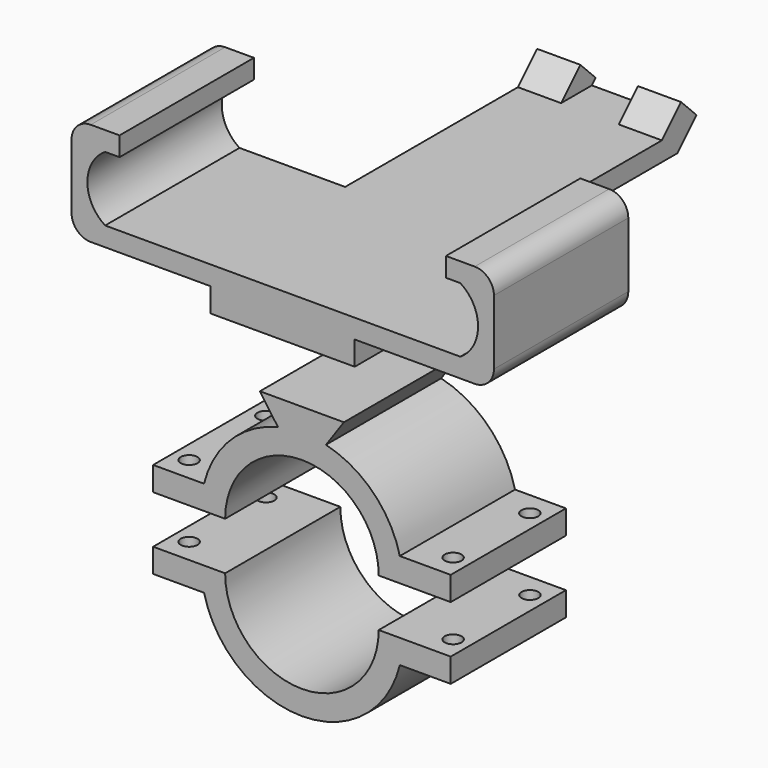
from build123d import *

# Parameters (mm, degrees)
F3_DEPTH      = 30
F4_DEPTH      = 5
F6_DEPTH      = 15
F6_DEPTH_BACK = 15
F7_DEPTH      = 6
F8_DEPTH      = 30
F9_DEPTH      = 30
F10_R         = 1.75
F11_DEPTH     = 50


# Not quite as in the source:
# - a feature names something its author has since deleted; it is built from what else it names


with BuildPart() as f3:
    # F2 (on offset) → F3 (new body)
    with BuildSketch(Plane.XZ.offset(30)):
        with BuildLine():
            Line((37, 49), (-37, 49))
            ThreePointArc((-37, 49), (-40.7061089907, 55.75), (-37, 62.5))
            Line((-37, 62.5), (-34, 62.5))
            Line((-34, 62.5), (-34, 66.5))
            Line((-34, 66.5), (-40, 66.5))
            ThreePointArc((-40, 66.5), (-42.8284271247, 65.3284271247), (-44, 62.5))
            Line((-44, 62.5), (-44, 49))
            ThreePointArc((-44, 49), (-42.8284271247, 46.1715728753), (-40, 45))
            Line((-40, 45), (-15, 45))
            Line((-15, 45), (-15, 40))
            Line((-15, 40), (-5.798962309, 40))
            Line((-5.798962309, 40), (-9.3, 45))
            Line((-9.3, 45), (9.3, 45))
            Line((9.3, 45), (5.798962309, 40))
            Line((5.798962309, 40), (15, 40))
            Line((15, 40), (15, 45))
            Line((15, 45), (40, 45))
            ThreePointArc((40, 45), (42.8284271247, 46.1715728753), (44, 49))
            Line((44, 49), (44, 62.5))
            ThreePointArc((44, 62.5), (42.8284271247, 65.3284271247), (40, 66.5))
            Line((40, 66.5), (34, 66.5))
            Line((34, 66.5), (34, 62.5))
            Line((34, 62.5), (37, 62.5))
            ThreePointArc((37, 62.5), (40.7061089907, 55.75), (37, 49))
        make_face()
    extrude(amount=-F3_DEPTH)

    # F2 (on offset) → F4 (join)
    with BuildSketch(Plane.XZ.offset(30)):
        with BuildLine():
            Line((37, 49), (-37, 49))
            ThreePointArc((-37, 49), (-40.7061089907, 55.75), (-37, 62.5))
            Line((-37, 62.5), (-34, 62.5))
            Line((-34, 62.5), (-34, 66.5))
            Line((-34, 66.5), (-40, 66.5))
            ThreePointArc((-40, 66.5), (-42.8284271247, 65.3284271247), (-44, 62.5))
            Line((-44, 62.5), (-44, 49))
            ThreePointArc((-44, 49), (-42.8284271247, 46.1715728753), (-40, 45))
            Line((-40, 45), (-15, 45))
            Line((-15, 45), (-15, 40))
            Line((-15, 40), (-5.798962309, 40))
            Line((-5.798962309, 40), (-9.3, 45))
            Line((-9.3, 45), (9.3, 45))
            Line((9.3, 45), (5.798962309, 40))
            Line((5.798962309, 40), (15, 40))
            Line((15, 40), (15, 45))
            Line((15, 45), (40, 45))
            ThreePointArc((40, 45), (42.8284271247, 46.1715728753), (44, 49))
            Line((44, 49), (44, 62.5))
            ThreePointArc((44, 62.5), (42.8284271247, 65.3284271247), (40, 66.5))
            Line((40, 66.5), (34, 66.5))
            Line((34, 66.5), (34, 62.5))
            Line((34, 62.5), (37, 62.5))
            ThreePointArc((37, 62.5), (40.7061089907, 55.75), (37, 49))
        make_face()
        Polygon((-9.3, 45), (-5.798962309, 40), (5.798962309, 40), (9.3, 45), align=None)
    extrude(amount=F4_DEPTH)

    # F5 (on Right) → F6 (join, two sides)
    with BuildSketch(Plane.YZ) as f6_sk:
        Polygon((45, 49), (0, 49), (0, 45), (49, 45), (53, 49), align=None)
        Polygon((50, 54), (45, 49), (53, 49), (54, 50), align=None)
    extrude(amount=F6_DEPTH)
    extrude(f6_sk.sketch, amount=-F6_DEPTH_BACK)

    # F5 (on Right) → F7 (cut, symmetric)
    with BuildSketch(Plane.YZ):
        Polygon((50, 54), (45, 49), (53, 49), (54, 50), align=None)
    extrude(amount=F7_DEPTH, both=True, mode=Mode.SUBTRACT)


with BuildPart() as f8:
    # F0 (on Front) → F8 (new body)
    with BuildSketch(Plane.XZ):
        with BuildLine():
            Line((-31, 0), (-21, 0))
            ThreePointArc((-21, 0), (-20.8484728355, 2.5181700556), (-20.3960780544, 5))
            Line((-20.3960780544, 5), (-31, 5))
            Line((-31, 5), (-31, 0))
        make_face()
        with BuildLine():
            Line((-21, 0), (-16, 0))
            Line((-16, 0), (-16, 5))
            Line((-16, 5), (-20.3960780544, 5))
            ThreePointArc((-20.3960780544, 5), (-20.8484728355, 2.5181700556), (-21, 0))
        make_face()
        with BuildLine():
            ThreePointArc((-16, 0), (0, 16), (16, 0))
            Line((16, 0), (16, 5))
            Line((16, 5), (20.3960780544, 5))
            ThreePointArc((20.3960780544, 5), (14.8492424049, 14.8492424049), (5, 20.3960780544))
            ThreePointArc((5, 20.3960780544), (0, 21), (-5, 20.3960780544))
            ThreePointArc((-5, 20.3960780544), (-14.8492424049, 14.8492424049), (-20.3960780544, 5))
            Line((-20.3960780544, 5), (-16, 5))
            Line((-16, 5), (-16, 0))
        make_face()
        with BuildLine():
            Line((16, 5), (16, 0))
            Line((16, 0), (21, 0))
            ThreePointArc((21, 0), (20.8484728355, 2.5181700556), (20.3960780544, 5))
            Line((20.3960780544, 5), (16, 5))
        make_face()
        with BuildLine():
            ThreePointArc((20.3960780544, 5), (20.8484728355, 2.5181700556), (21, 0))
            Line((21, 0), (31, 0))
            Line((31, 0), (31, 5))
            Line((31, 5), (20.3960780544, 5))
        make_face()
        with BuildLine():
            ThreePointArc((-5, 20.3960780544), (0, 21), (5, 20.3960780544))
            Line((5, 20.3960780544), (8.75, 25.7516330797))
            Line((8.75, 25.7516330797), (-8.75, 25.7516330797))
            Line((-8.75, 25.7516330797), (-5, 20.3960780544))
        make_face()
    extrude(amount=F8_DEPTH)


with BuildPart() as f9:
    # F0 (on Front) → F9 (new body)
    with BuildSketch(Plane.XZ):
        with BuildLine():
            ThreePointArc((-20.3960780544, -15), (-20.8484728355, -12.5181700556), (-21, -10))
            Line((-21, -10), (-31, -10))
            Line((-31, -10), (-31, -15))
            Line((-31, -15), (-20.3960780544, -15))
        make_face()
        with BuildLine():
            Line((-16, -15), (-16, -10))
            Line((-16, -10), (-21, -10))
            ThreePointArc((-21, -10), (-20.8484728355, -12.5181700556), (-20.3960780544, -15))
            Line((-20.3960780544, -15), (-16, -15))
        make_face()
        with BuildLine():
            ThreePointArc((16, -10), (0, -26), (-16, -10))
            Line((-16, -10), (-16, -15))
            Line((-16, -15), (-20.3960780544, -15))
            ThreePointArc((-20.3960780544, -15), (0, -31), (20.3960780544, -15))
            Line((20.3960780544, -15), (16, -15))
            Line((16, -15), (16, -10))
        make_face()
        with BuildLine():
            Line((21, -10), (16, -10))
            Line((16, -10), (16, -15))
            Line((16, -15), (20.3960780544, -15))
            ThreePointArc((20.3960780544, -15), (20.8484728355, -12.5181700556), (21, -10))
        make_face()
        with BuildLine():
            Line((31, -10), (21, -10))
            ThreePointArc((21, -10), (20.8484728355, -12.5181700556), (20.3960780544, -15))
            Line((20.3960780544, -15), (31, -15))
            Line((31, -15), (31, -10))
        make_face()
    extrude(amount=F9_DEPTH)


with BuildPart() as f11_tool:
    # F10 (on face) → F11 (new body)
    with BuildSketch(Plane.XY.offset(5)):
        with Locations((-27.5, -25)):
            Circle(F10_R)
        with Locations((-27.5, -5)):
            Circle(F10_R)
        with Locations((27.5, -5)):
            Circle(F10_R)
        with Locations((27.5, -25)):
            Circle(F10_R)
    extrude(amount=-F11_DEPTH)


with BuildPart() as f8_1:
    add(f8.part)

    # F11: cut by f11_tool
    add(f11_tool.part, mode=Mode.SUBTRACT)


with BuildPart() as f9_1:
    add(f9.part)

    # F11: cut by f11_tool
    add(f11_tool.part, mode=Mode.SUBTRACT)


solid = Compound([f3.part, f8_1.part, f9_1.part])
